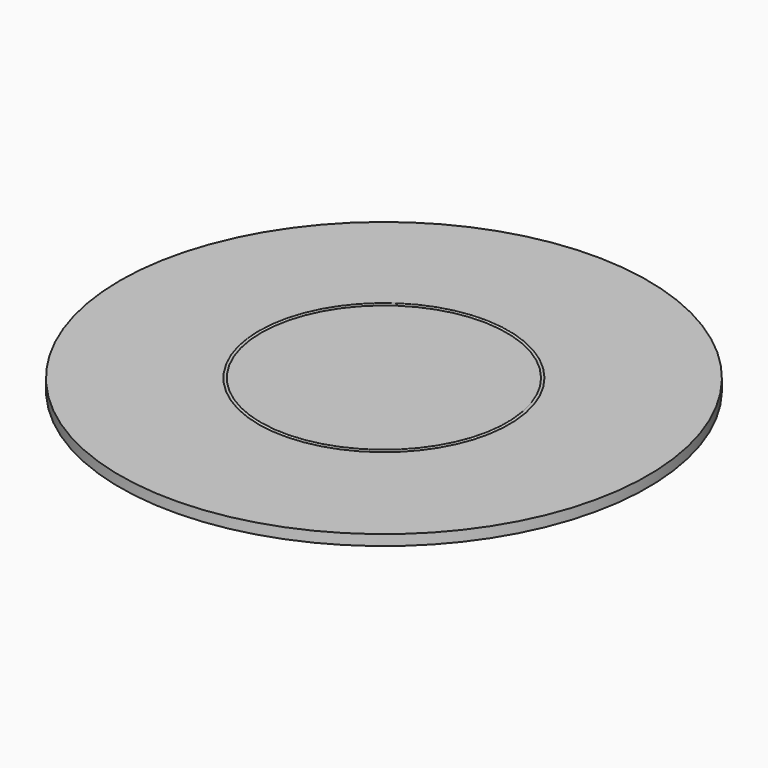
from build123d import *


# Not quite as in the source:
# - the program builds the solid bodies; features that only make, move or delete a surface that nothing else refers to are left out


with BuildPart() as f1:
    # F0 (on Front) → F1 (revolve)
    with BuildSketch(Plane.XZ):
        Polygon((262.5, 0), (0, 0), (0, -20), (500, -20), (500, 0), (267.5, 0), align=None)
        with BuildLine():
            ThreePointArc((267.5, 0), (265, 2.5), (262.5, 0))
            Line((262.5, 0), (267.5, 0))
        make_face()
    revolve(axis=Axis((500, 0, -10), (0, 0, -1)))


solid = f1.part
